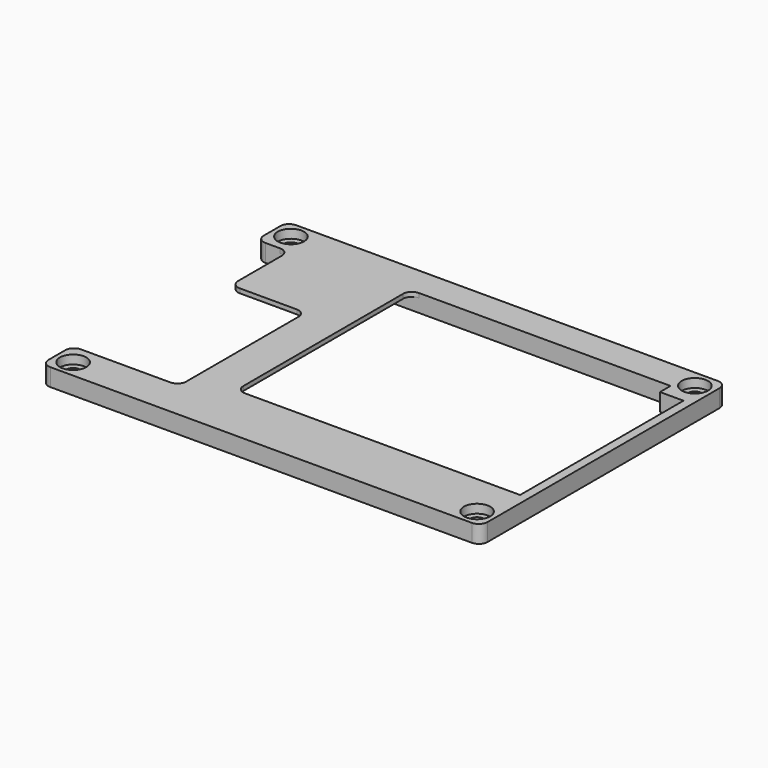
from build123d import *

# Parameters (mm, degrees)
F0_W     = 100
F0_H     = 70
F1_DEPTH = 4
F2_R     = 1.65
F3_DEPTH = 4
F2_W     = 17
F2_H     = 36
F2_W_2   = 59.3
F2_H_2   = 3
F4_DEPTH = 4
F6_DEPTH = 3
F7_R     = 3
F8_DEPTH = 2
F9_R     = 2


with BuildPart() as f1:
    # F0 (on Top) → F1 (new body)
    with BuildSketch(Plane.XY):
        Rectangle(F0_W, F0_H)
    extrude(amount=F1_DEPTH)

    # F2 (on face) → F3 (cut, through all)
    with BuildSketch(Plane.XY.offset(4)):
        with Locations((-46, 31)):
            Circle(F2_R)
        with Locations((46, 31)):
            Circle(F2_R)
        with Locations((46, -31)):
            Circle(F2_R)
        with Locations((-46, -31)):
            Circle(F2_R)
    extrude(amount=-F3_DEPTH, mode=Mode.SUBTRACT)

    # F2 (on face) → F4 (cut, through all)
    with BuildSketch(Plane.XY.offset(4)):
        with Locations((-34.15, -8.25)):
            Rectangle(F2_W, F2_H)
        Polygon((-42.65, -26.25), (-42.65, 9.75), (-42.65, 26.25), (-50, 26.25), (-50, -26.25), align=None)
        with Locations((13, 26.75)):
            Rectangle(F2_W_2, F2_H_2)
        Polygon((42.65, 25.25), (-16.65, 25.25), (-16.65, -21.25), (-15, -21.25), (35, -21.25), (42.65, -21.25), (48, -21.25), (48, 25.25), align=None)
    extrude(amount=-F4_DEPTH, mode=Mode.SUBTRACT)

    # F5 (on face) → F6 (cut)
    with BuildSketch(Plane.XY):
        Polygon((-50, -26.25), (-22.65, -26.25), (-22.65, -28.25), (-15, -28.25), (-15, -21.25), (35, -21.25), (35, -28.25), (42.65, -28.25), (42.65, -21.25), (48, -21.25), (48, 25.25), (42.65, 25.25), (42.65, 28.25), (-22.65, 28.25), (-22.65, 26.25), (-50, 26.25), align=None)
    extrude(amount=F6_DEPTH, mode=Mode.SUBTRACT)

    # F7 (on face) → F8 (cut)
    with BuildSketch(Plane.XY.offset(4)):
        with Locations((-46, 31)):
            Circle(F7_R)
        with Locations((46, 31)):
            Circle(F7_R)
        with Locations((46, -31)):
            Circle(F7_R)
        with Locations((-46, -31)):
            Circle(F7_R)
    extrude(amount=-F8_DEPTH, mode=Mode.SUBTRACT)

    # F9
    f9_edges = [f1.edges().sort_by_distance(p)[0] for p in [
        (-50, 35, 2),
        (-50, -35, 2),
        (50, -35, 2),
        (50, 35, 2),
        (-16.65, -21.25, 3.5),
        (-16.65, 28.25, 3.5),
        (-50, 26.25, 2),
        (-50, -26.25, 2),
        (-42.65, 26.25, 3.5),
        (-42.65, 9.75, 3.5),
        (-25.65, 9.75, 3.5),
        (-25.65, -26.25, 3.5),
    ]]
    fillet(f9_edges, radius=F9_R)


solid = f1.part
